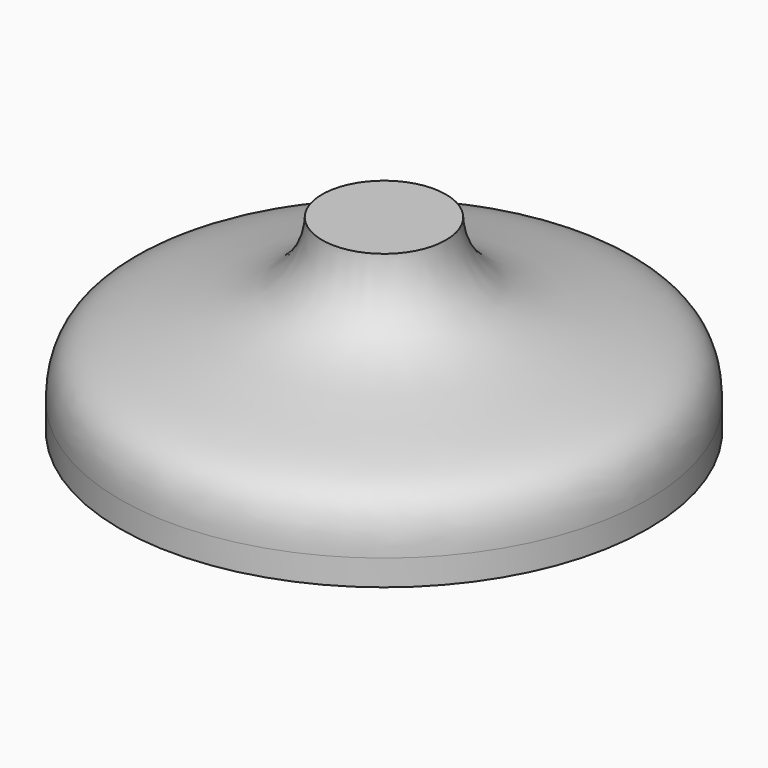
from build123d import *


# Not quite as in the source:
# - the program builds the solid bodies; features that only make, move or delete a surface that nothing else refers to are left out


with BuildPart() as f3:
    # F2 (on Front) → F3 (revolve)
    with BuildSketch(Plane.XZ):
        with BuildLine():
            Line((0, 0), (73.025, 0))
            Line((73.025, 0), (73.025, 7.112))
            add(Edge.make_bspline(
                [(73.025, 7.112), (73.015047562, 10.8343630777), (72.2485598093, 15.8945775164), (66.3275190936, 24.9686965772), (31.2000310376, 29.0237063536), (19.0448345768, 41.1321634463), (17.1791362136, 48.9114817586), (17.1172395349, 52.0846992731)],
                knots=[0, 0, 0, 0, 0.1547394037, 0.3126165344, 0.6193609099, 0.8331037231, 1, 1, 1, 1], degree=3))
            Line((17.1172395349, 52.0846992731), (0, 52.0846992731))
            Line((0, 52.0846992731), (0, 0))
        make_face()
    revolve(axis=Axis((0, 0, 26.0423496366), (0, 0, -1)))


solid = f3.part
